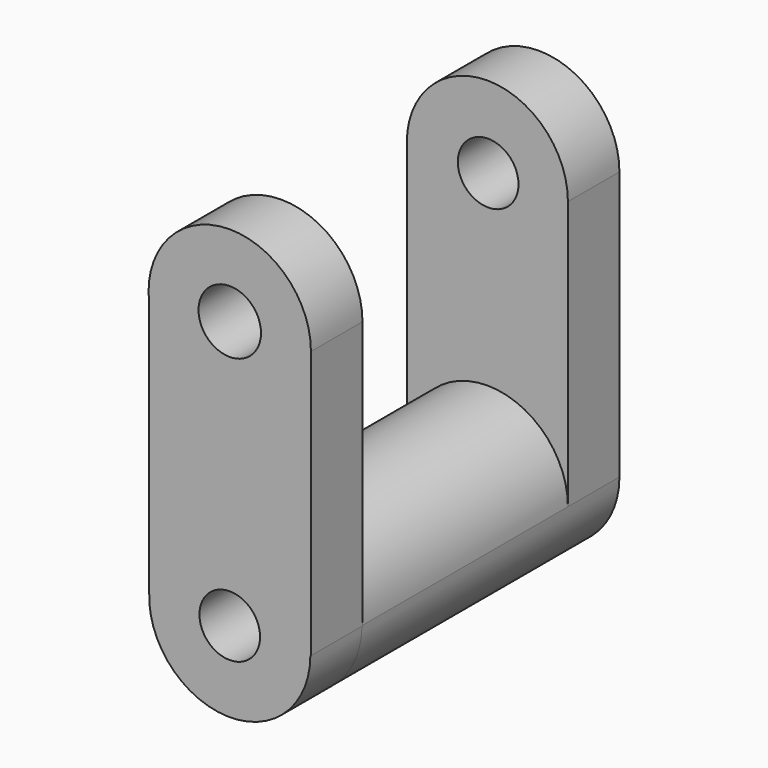
from build123d import *

# Parameters (mm, degrees)
F0_R     = 8.9668874309
F1_DEPTH = 19.05
F2_R     = 8.9668874309
F3_DEPTH = 76.2
F4_R     = 9.2392486584
F5_DEPTH = 19.05
F6_DEPTH = 19.05


with BuildPart() as f1:
    # F0 (on Front) → F1 (new body)
    with BuildSketch(Plane.XZ):
        with BuildLine():
            Line((-23.8205983585, 48.6063640565), (-23.8205983585, -30.8263637125))
            ThreePointArc((-23.8205983585, -30.8263637125), (0, -54.6469620711), (23.8205983585, -30.8263637125))
            Line((23.8205983585, -30.8263637125), (23.8205983585, 48.6063640565))
            ThreePointArc((23.8205983585, 48.6063640565), (0, 72.426962415), (-23.8205983585, 48.6063640565))
        make_face()
        with Locations((0, -30.8263637125)):
            Circle(F0_R, mode=Mode.SUBTRACT)
        with Locations((0.2309088741, 48.3754538)):
            Circle(F0_R, mode=Mode.SUBTRACT)
    extrude(amount=F1_DEPTH)

    # F2 (on face) → F3 (join)
    with BuildSketch(Plane.XZ.offset(19.05)):
        with BuildLine():
            ThreePointArc((-23.8205983585, -30.8263637125), (0, -54.6469620711), (23.8205983585, -30.8263637125))
            ThreePointArc((23.8205983585, -30.8263637125), (0, -7.005765354), (-23.8205983585, -30.8263637125))
        make_face()
        with Locations((0, -30.8263637125)):
            Circle(F2_R, mode=Mode.SUBTRACT)
    extrude(amount=F3_DEPTH)

    # F4 (on face) → F5 (join)
    with BuildSketch(Plane.XZ.offset(95.25)):
        with BuildLine():
            Line((-23.8205983585, 45.3295558312), (-23.8205983585, -29.759446989))
            ThreePointArc((-23.8205983585, -29.759446989), (-0.5335919833, -54.6648724127), (23.8444798109, -30.8263637125))
            Line((23.8444798109, -30.8263637125), (24.0145456046, -30.8263637125))
            Line((24.0145456046, -30.8263637125), (24.0145456046, 48.3754538))
            ThreePointArc((24.0145456046, 48.3754538), (-1.5260332541, 72.3414635451), (-23.8205983585, 45.3295558312))
        make_face()
        with BuildLine():
            ThreePointArc((23.8205983585, -30.8263637125), (0, -54.6469620711), (-23.8205983585, -30.8263637125))
            ThreePointArc((-23.8205983585, -30.8263637125), (0, -7.005765354), (23.8205983585, -30.8263637125))
        make_face(mode=Mode.SUBTRACT)
        with Locations((0, 48.3754538)):
            Circle(F4_R, mode=Mode.SUBTRACT)
    extrude(amount=F5_DEPTH)

    # F6 (add): a face of the model
    f6_faces = [f1.faces().sort_by_distance(p)[0] for p in [
        (-23.1468500933, -95.25, -30.8263637125),
    ]]
    extrude(f6_faces, amount=F6_DEPTH)


solid = f1.part
